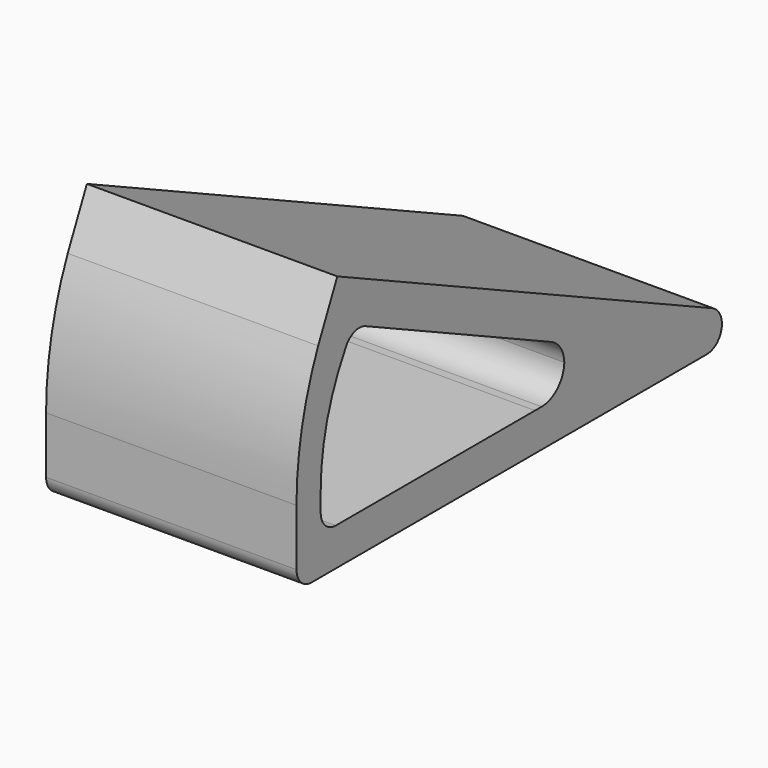
from build123d import *

# Parameters (mm, degrees)
F1_DEPTH    = 13.25
F2_DEPTH    = 13.25
F3_R        = 1.99999
F4_R        = 2
F5_T1_DEPTH = 26.5


# Not quite as in the source:
# - a fillet or chamfer that OpenCascade refuses, or shapes differently, is made with other operations: its cross-section is extruded or revolved along the edge and cut away or added
# - a fillet or chamfer is up to 0.001 mm smaller than in the source, because OpenCascade refuses the exact size
# - a feature names something its author has since deleted; it is built from what else it names


with BuildPart() as f1:
    # F0 (on Right) → F1 (new body, symmetric)
    with BuildSketch(Plane.YZ):
        with BuildLine():
            Line((24.6479697927, -2.219830174), (-24.9527402653, 20.909360776))
            Line((-24.9527402653, 20.909360776), (-27.4884498358, 15.4715140538))
            Line((-27.4884498358, 15.4715140538), (-23.8632186876, 13.7810410068))
            Line((-23.8632186876, 13.7810410068), (-23.0179821641, 15.5936565809))
            Line((-23.0179821641, 15.5936565809), (5.077559234, 2.4924904669))
            Line((5.077559234, 2.4924904669), (7.7964825951, 1.2246356817))
            Line((7.7964825951, 1.2246356817), (15.1652631053, -2.2114831015))
            Line((15.1652631053, -2.2114831015), (5.077559234, -2.2175114543))
            Line((5.077559234, -2.2175114543), (1.1974681402, -2.219830174))
            Line((1.1974681402, -2.219830174), (-27.1520302073, -2.219830174))
            Line((-27.1520302073, -2.219830174), (-27.1520302073, 1.780169826))
            Line((-27.1520302073, 1.780169826), (-30.3520302073, 1.780169826))
            Line((-30.3520302073, 1.780169826), (-30.3520302073, -6.219830174))
            Line((-30.3520302073, -6.219830174), (24.6479697927, -6.219830174))
            ThreePointArc((24.6479697927, -6.219830174), (25.9221103143, -4.219830174), (24.6479697927, -2.219830174))
        make_face()
        with BuildLine():
            Line((-23.8632186876, 13.7810410068), (-27.4884498358, 15.4715140538))
            ThreePointArc((-27.4884498358, 15.4715140538), (-29.6284726398, 8.7739706401), (-30.3520302073, 1.780169826))
            Line((-30.3520302073, 1.780169826), (-27.1520302073, 1.780169826))
            ThreePointArc((-27.1520302073, 1.780169826), (-26.3149438564, 8.0018494688), (-23.8632186876, 13.7810410068))
        make_face()
        Polygon((7.7964825951, 1.2246356817), (5.077559234, 2.4924904669), (5.077559234, -2.2175114543), (15.1652631053, -2.2114831015), align=None)
    extrude(amount=F1_DEPTH, both=True)

    # F0 (on Right) → F2 (join, symmetric)
    with BuildSketch(Plane.YZ):
        with BuildLine():
            Line((24.6479697927, -2.219830174), (-24.9527402653, 20.909360776))
            Line((-24.9527402653, 20.909360776), (-27.4884498358, 15.4715140538))
            Line((-27.4884498358, 15.4715140538), (-23.8632186876, 13.7810410068))
            Line((-23.8632186876, 13.7810410068), (-23.0179821641, 15.5936565809))
            Line((-23.0179821641, 15.5936565809), (5.077559234, 2.4924904669))
            Line((5.077559234, 2.4924904669), (7.7964825951, 1.2246356817))
            Line((7.7964825951, 1.2246356817), (15.1652631053, -2.2114831015))
            Line((15.1652631053, -2.2114831015), (5.077559234, -2.2175114543))
            Line((5.077559234, -2.2175114543), (1.1974681402, -2.219830174))
            Line((1.1974681402, -2.219830174), (-27.1520302073, -2.219830174))
            Line((-27.1520302073, -2.219830174), (-27.1520302073, 1.780169826))
            Line((-27.1520302073, 1.780169826), (-30.3520302073, 1.780169826))
            Line((-30.3520302073, 1.780169826), (-30.3520302073, -6.219830174))
            Line((-30.3520302073, -6.219830174), (24.6479697927, -6.219830174))
            ThreePointArc((24.6479697927, -6.219830174), (25.9221103143, -4.219830174), (24.6479697927, -2.219830174))
        make_face()
    extrude(amount=F2_DEPTH, both=True)

    # F3 (radius 2 in the source; OpenCascade refuses exactly that, so slightly less here)
    f3_edges = [f1.edges().sort_by_distance(p)[0] for p in [
        (0, -23.017982, 15.593657),
        (0, 24.64797, -2.21983),
        (0, 24.64797, -6.21983),
    ]]
    fillet(f3_edges, radius=F3_R)

    # F4
    f4_edges = [f1.edges().sort_by_distance(p)[0] for p in [
        (0, -27.15203, -2.21983),
        (0, -30.35203, -6.21983),
        (0, -30.35203, 1.78017),
    ]]
    fillet(f4_edges, radius=F4_R)

    # F5: fillet of radius 3 on 2 edges, made by hand

    # F5_s2 → F5_t1 (join)
    with BuildSketch(Plane.YZ.offset(-13.25)):
        with BuildLine():
            ThreePointArc((2.0793520161, -2.2193031654), (4.1995133271, -1.3399901057), (5.077559234, 0.780696299))
            Line((5.077559234, 0.780696299), (5.077559234, -2.2175114543))
            Line((5.077559234, -2.2175114543), (2.0793520161, -2.2193031654))
        make_face()
        with BuildLine():
            ThreePointArc((5.077559234, 0.5812796845), (4.6077335715, 2.1931785095), (3.3454140192, 3.3002030456))
            Line((3.3454140192, 3.3002030456), (5.077559234, 2.4924904669))
            Line((5.077559234, 2.4924904669), (5.077559234, 0.5812796845))
        make_face()
    extrude(amount=F5_T1_DEPTH)


solid = f1.part
